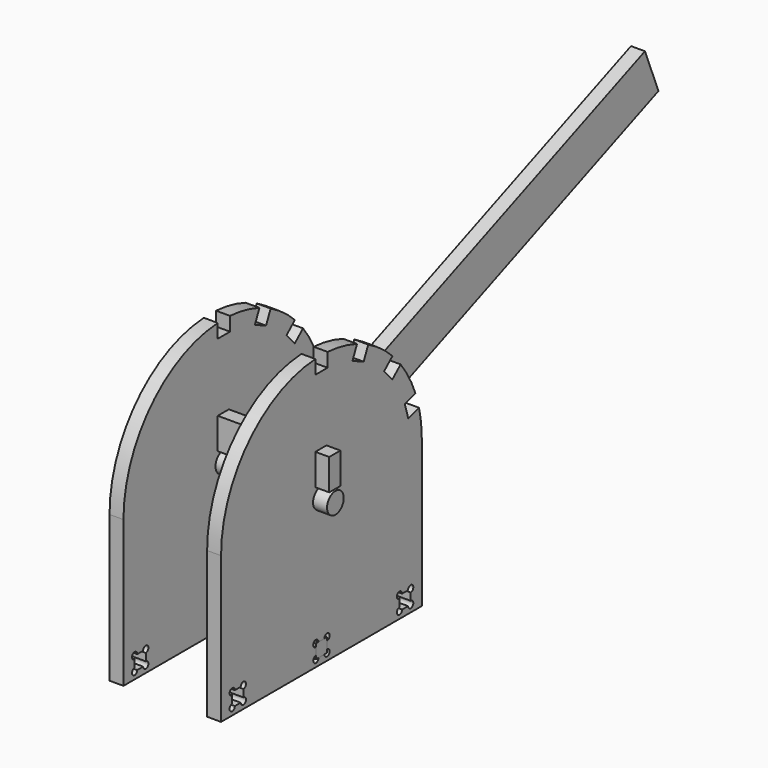
from build123d import *

# Parameters (mm, degrees)
F3_R           = 9.525
F4_DEPTH       = 12.7
F6_R           = 9.525
F7_DEPTH       = 63.5
F7_DEPTH_BACK  = 63.5
F9_DEPTH       = 12.7
F11_DEPTH      = 12.7
F12_R          = 6.35
F12_R_2        = 18.8468
F13_DEPTH      = 6.35
F13_DEPTH_BACK = 6.35


# Not quite as in the source:
# - a feature names something its author has since deleted; it is built from what else it names


with BuildPart() as f4:
    # F3 (on offset) → F4 (new body)
    with BuildSketch(Plane.YZ.offset(38.1)):
        with BuildLine():
            Line((-114.3, 127), (-114.3, -6.35))
            Line((-114.3, -6.35), (114.3, -6.35))
            Line((114.3, -6.35), (114.3, 127))
            ThreePointArc((114.3, 127), (113.4875193986, 140.6041515996), (111.0616283334, 154.0148979626))
            Line((111.0616283334, 154.0148979626), (98.9279460754, 150.2647306514))
            Line((98.9279460754, 150.2647306514), (94.802762033, 163.6117811352))
            Line((94.802762033, 163.6117811352), (106.936444291, 167.3619484464))
            ThreePointArc((106.936444291, 167.3619484464), (99.6654310495, 182.9579471899), (90.1355302257, 197.2856755742))
            Line((90.1355302257, 197.2856755742), (80.6164381776, 188.8787209188))
            Line((80.6164381776, 188.8787209188), (71.3687880566, 199.3497221717))
            Line((71.3687880566, 199.3497221717), (80.8878801047, 207.7566768272))
            ThreePointArc((80.8878801047, 207.7566768272), (67.8479656545, 218.9844745408), (53.2702970855, 228.1274712846))
            Line((53.2702970855, 228.1274712846), (48.0491058481, 216.5503748411))
            Line((48.0491058481, 216.5503748411), (35.3142997602, 222.2936852023))
            Line((35.3142997602, 222.2936852023), (40.5354909977, 233.8707816458))
            ThreePointArc((40.5354909977, 233.8707816458), (24.0325912935, 238.7449084107), (6.985, 241.0863698038))
            Line((6.985, 241.0863698038), (6.985, 228.3863698038))
            Line((6.985, 228.3863698038), (-6.985, 228.3863698038))
            Line((-6.985, 228.3863698038), (-6.985, 241.0863698038))
            ThreePointArc((-6.985, 241.0863698038), (-83.2552565908, 205.3138062541), (-114.3, 127))
        make_face()
        with BuildLine():
            ThreePointArc((-98.6, 0), (-103.7213203436, -2.1213203436), (-101.6, 3))
            Line((-101.6, 3), (-101.6, 9.7))
            ThreePointArc((-101.6, 9.7), (-103.7213203436, 14.8213203436), (-98.6, 12.7))
            Line((-98.6, 12.7), (-91.9, 12.7))
            ThreePointArc((-91.9, 12.7), (-86.7786796564, 14.8213203436), (-88.9, 9.7))
            Line((-88.9, 9.7), (-88.9, 3))
            ThreePointArc((-88.9, 3), (-86.7786796564, -2.1213203436), (-91.9, 0))
            Line((-91.9, 0), (-98.6, 0))
        make_face(mode=Mode.SUBTRACT)
        with BuildLine():
            ThreePointArc((-3.35, 0), (-8.4713203436, -2.1213203436), (-6.35, 3))
            Line((-6.35, 3), (-6.35, 9.7))
            ThreePointArc((-6.35, 9.7), (-8.4713203436, 14.8213203436), (-3.35, 12.7))
            Line((-3.35, 12.7), (3.35, 12.7))
            ThreePointArc((3.35, 12.7), (8.4713203436, 14.8213203436), (6.35, 9.7))
            Line((6.35, 9.7), (6.35, 3))
            ThreePointArc((6.35, 3), (8.4713203436, -2.1213203436), (3.35, 0))
            Line((3.35, 0), (-3.35, 0))
        make_face(mode=Mode.SUBTRACT)
        with BuildLine():
            Line((101.6, 9.7), (101.6, 3))
            ThreePointArc((101.6, 3), (103.7213203436, -2.1213203436), (98.6, 0))
            Line((98.6, 0), (91.9, 0))
            ThreePointArc((91.9, 0), (86.7786796564, -2.1213203436), (88.9, 3))
            Line((88.9, 3), (88.9, 9.7))
            ThreePointArc((88.9, 9.7), (86.7786796564, 14.8213203436), (91.9, 12.7))
            Line((91.9, 12.7), (98.6, 12.7))
            ThreePointArc((98.6, 12.7), (103.7213203436, 14.8213203436), (101.6, 9.7))
        make_face(mode=Mode.SUBTRACT)
        with Locations((0, 127)):
            Circle(F3_R, mode=Mode.SUBTRACT)
    extrude(amount=F4_DEPTH)


with BuildPart() as f5_1:
    # F5: instance of F4
    add(f4.part.mirror(Plane.YZ))


with BuildPart() as f7:
    # F6 (on Right) → F7 (new body, two sides)
    with BuildSketch(Plane.YZ) as f7_sk:
        with Locations((0, 127)):
            Circle(F6_R)
    extrude(amount=F7_DEPTH)
    extrude(f7_sk.sketch, amount=-F7_DEPTH_BACK)


with BuildPart() as f9:
    # F8 (on Top) → F9 (new body)
    with BuildSketch(Plane.XY):
        Polygon((-38.1, -6.35), (-38.1, -12.7), (38.1, -12.7), (38.1, -6.35), (50.8, -6.35), (50.8, 6.35), (38.1, 6.35), (38.1, 12.7), (-38.1, 12.7), (-38.1, 6.35), (-50.8, 6.35), (-50.8, -6.35), align=None)
    extrude(amount=F9_DEPTH)


with BuildPart() as f11:
    # F10 (on face) → F11 (new body)
    with BuildSketch(Plane(origin=(0, -6.985, 0), x_dir=(-1, 0, 0), z_dir=(0, 1, 0))):
        Polygon((38.1, 138.2272196057), (38.1, 153.9272196057), (50.8, 153.9272196057), (50.8, 138.2272196057), (63.5, 138.2272196057), (63.5, 166.6272196057), (-63.5, 166.6272196057), (-63.5, 138.2272196057), (-50.8, 138.2272196057), (-50.8, 153.9272196057), (-36.83, 153.9272196057), (-36.83, 138.2272196057), align=None)
    extrude(amount=F11_DEPTH)


with BuildPart() as f13:
    # F12 (on Right) → F13 (new body, two sides)
    with BuildSketch(Plane.YZ) as f13_sk:
        with BuildLine():
            Line((439.3304503869, 260.0993646615), (423.9084583079, 298.2701345098))
            Line((423.9084583079, 298.2701345098), (70.651409718, 155.5450224183))
            ThreePointArc((70.651409718, 155.5450224183), (52.6775037256, 152.9509477861), (35.5445156861, 158.9718481058))
            ThreePointArc((35.5445156861, 158.9718481058), (12.7005316335, 166.9997151987), (-11.2646763564, 163.5409490225))
            Line((-11.2646763564, 163.5409490225), (-26.0477461621, 157.5682011226))
            ThreePointArc((-26.0477461621, 157.5682011226), (-39.5731561265, 144.7088099424), (-40.659802818, 126.0776571279))
            ThreePointArc((-40.659802818, 126.0776571279), (-40.8771321563, 122.351426565), (-43.5822141492, 119.779548329))
            Line((-43.5822141492, 119.779548329), (-44.6488614796, 119.3485948338))
            ThreePointArc((-44.6488614796, 119.3485948338), (-51.5817693821, 112.5356452126), (-51.6665926962, 102.8158561444))
            ThreePointArc((-51.6665926962, 102.8158561444), (-44.853643075, 95.8829482419), (-35.1338540068, 95.7981249278))
            Line((-35.1338540068, 95.7981249278), (-33.561058403, 96.4335755996))
            ThreePointArc((-33.561058403, 96.4335755996), (-30.0711457165, 96.549257501), (-27.3310085278, 94.3848820601))
            ThreePointArc((-27.3310085278, 94.3848820601), (-13.6303225842, 83.5630048559), (3.8192408484, 84.1414143627))
            Line((3.8192408484, 84.1414143627), (439.3304503869, 260.0993646615))
        make_face()
        with Locations((-39.8913577432, 107.5733598808)):
            Circle(F12_R, mode=Mode.SUBTRACT)
        with Locations((0, 127)):
            Circle(F12_R_2, mode=Mode.SUBTRACT)
    extrude(amount=F13_DEPTH)
    extrude(f13_sk.sketch, amount=-F13_DEPTH_BACK)


solid = Compound([f4.part, f5_1.part, f7.part, f9.part, f11.part, f13.part])
